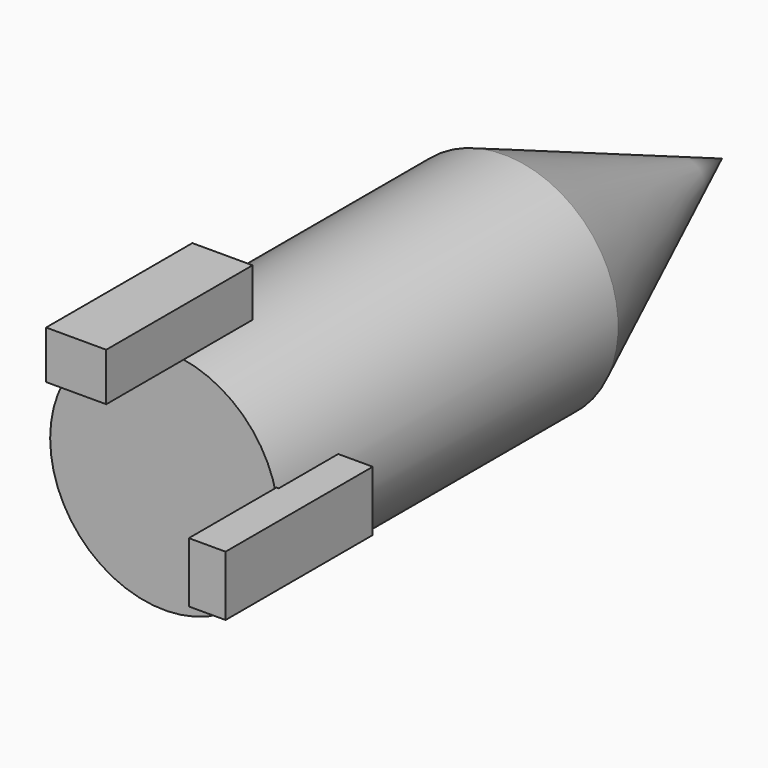
from build123d import *

# Parameters (mm, degrees)
F4_DEPTH  = 356.7984104156
F0_R      = 96.474269749
F5_DEPTH  = 358.334004879
F7_W      = 31.0177132487
F7_H      = 155.3362011909
F9_DEPTH  = 25.4
F10_DEPTH = 25.4
F8_W      = 155.1911532879
F8_H      = 39.4811406732
F11_DEPTH = 25.4
F12_DEPTH = 25.4
F7_W_2    = 35.9391272068
F7_H_2    = 158.800393343
F13_DEPTH = 25.4
F14_DEPTH = 25.4
F15_DEPTH = 25.4
F8_W_2    = 154.4083654881
F8_H_2    = 40.5437201262
F16_DEPTH = 25.4
F17_DEPTH = 25.4
F5_FACE_R = 96.474269749


with BuildPart() as f4:
    # F3 (on face) → F4 (new body)
    with BuildSketch(Plane.XZ):
        with BuildLine():
            ThreePointArc((96.474269749, 0), (0, 96.474269749), (-96.474269749, 0))
            Line((-96.474269749, 0), (0, 0))
            Line((0, 0), (96.474269749, 0))
        make_face()
    extrude(amount=F4_DEPTH)

    # F0 (on Front) → F5 (join)
    with BuildSketch(Plane.XZ):
        Circle(F0_R)
    extrude(amount=F5_DEPTH)

    # F7 (on Top) → F9 (join)
    with BuildSketch(Plane.XY):
        with Locations((-110.0929714739, -373.1260895729)):
            Rectangle(F7_W, F7_H)
    extrude(amount=-F9_DEPTH)

    # F10 (add): a face of the model
    f10_faces = [f4.faces().sort_by_distance(p)[0] for p in [
        (-110.4612875771, -374.2952426729, 0),
    ]]
    extrude(f10_faces, amount=F10_DEPTH)


with BuildPart() as f11:
    # F8 (on Right) → F11 (new body)
    with BuildSketch(Plane.YZ):
        with Locations((-374.6730536222, -119.7640411556)):
            Rectangle(F8_W, F8_H)
    extrude(amount=-F11_DEPTH)

    # F12 (add): a face of the model
    f12_faces = [f11.faces().sort_by_distance(p)[0] for p in [
        (0, -374.6730536222, -119.7640411556),
    ]]
    extrude(f12_faces, amount=F12_DEPTH)


with BuildPart() as f13:
    # F7 (on Top) → F13 (new body)
    with BuildSketch(Plane.XY):
        with Locations((116.1221414804, -374.288007617)):
            Rectangle(F7_W_2, F7_H_2)
    extrude(amount=F13_DEPTH)

    # F7 (on Top) → F14 (join)
    with BuildSketch(Plane.XY):
        with Locations((116.1221414804, -374.288007617)):
            Rectangle(F7_W_2, F7_H_2)
    extrude(amount=F14_DEPTH)

    # F7 (on Top) → F15 (join)
    with BuildSketch(Plane.XY):
        with Locations((116.1221414804, -374.288007617)):
            Rectangle(F7_W_2, F7_H_2)
    extrude(amount=-F15_DEPTH)


with BuildPart() as f16:
    # F8 (on Right) → F16 (new body)
    with BuildSketch(Plane.YZ):
        with Locations((-374.2816597223, 122.9500994086)):
            Rectangle(F8_W_2, F8_H_2)
    extrude(amount=F16_DEPTH)

    # F8 (on Right) → F17 (join)
    with BuildSketch(Plane.YZ):
        with Locations((-374.2816597223, 122.9500994086)):
            Rectangle(F8_W_2, F8_H_2)
    extrude(amount=-F17_DEPTH)


with BuildPart() as f19:
    # F5_face (on face) → F19 section 0
    with BuildSketch(Plane(origin=(0, 0, 0), x_dir=(-1, 0, 0), z_dir=(0, 1, 0)), mode=Mode.PRIVATE) as f19_s0:
        Circle(F5_FACE_R)
    loft([Vertex(0, 230.1296591759, 0), f19_s0.sketch])


with BuildPart() as f20_1:
    # F20: instance of F4
    add(f4.part.mirror(Plane.YZ))


solid = Compound([f16.part, f19.part, f20_1.part])
